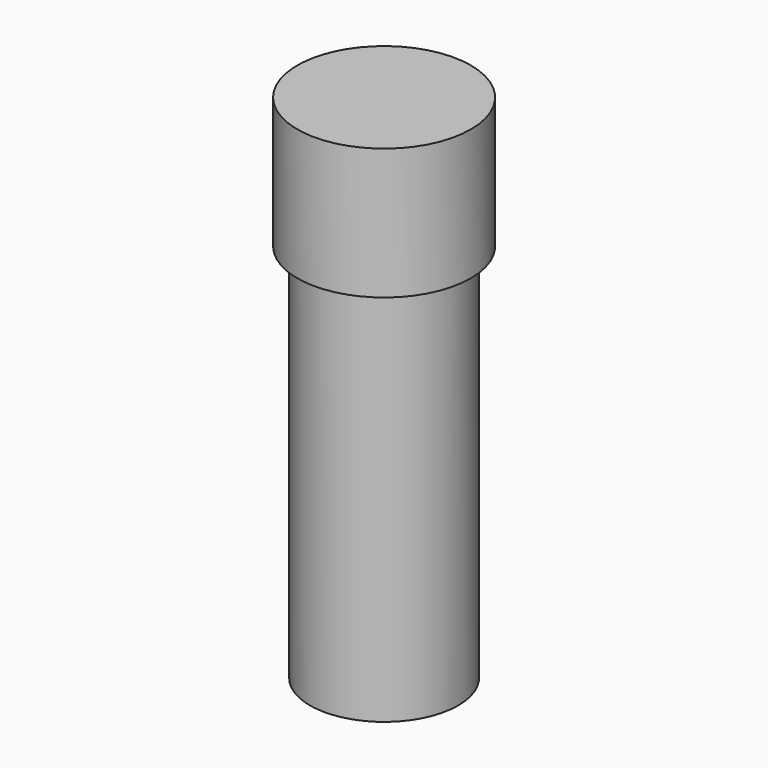
from build123d import *

# Parameters (mm, degrees)
F0_R     = 3.97
F0_R_2   = 3.108
F1_DEPTH = 6
F2_R     = 3.395
F3_DEPTH = 17.4


# Not quite as in the source:
# - a feature names something its author has since deleted; it is built from what else it names


with BuildPart() as f1:
    # F0 (on Top) → F1 (new body)
    with BuildSketch(Plane.XY):
        with Locations((-39.6077372134, 50.8700013161)):
            Circle(F0_R)
        with Locations((-39.6077372134, 50.8700013161)):
            Circle(F0_R_2, mode=Mode.SUBTRACT)
        with Locations((-39.6077372134, 50.8700013161)):
            Circle(F0_R_2)
    extrude(amount=F1_DEPTH)

    # F2 (on face) → F3 (join)
    with BuildSketch(Plane(origin=(0, 0, 0), x_dir=(1, 0, 0), z_dir=(0, 0, -1))):
        with Locations((-39.6077372134, -50.8700013161)):
            Circle(F2_R)
    extrude(amount=F3_DEPTH)


solid = f1.part
